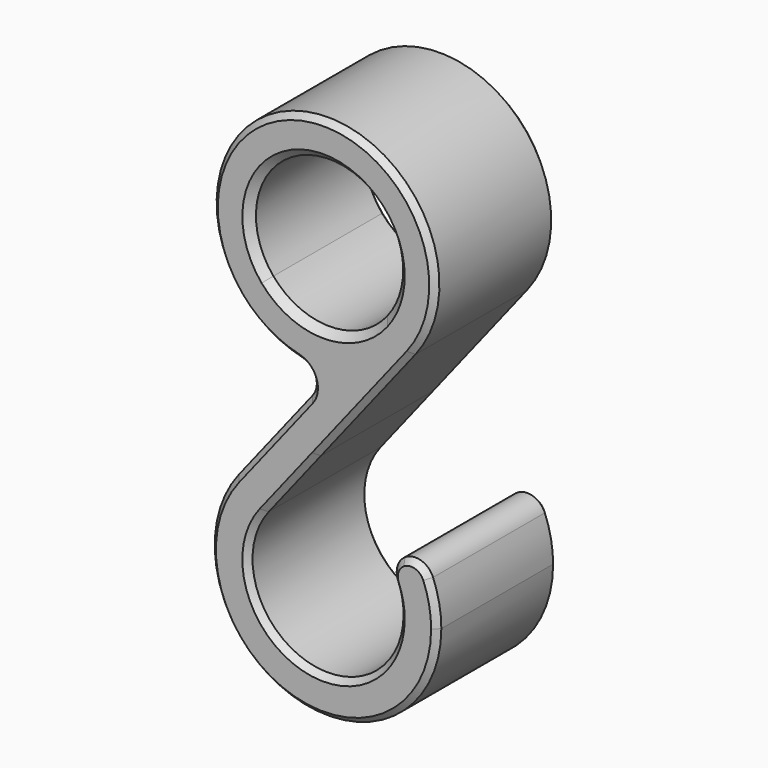
from build123d import *

# Parameters (mm, degrees)
F1_DEPTH = 16
F2_R     = 1.99999
F3_SIZE  = 0.8
F4_SIZE  = 0.6


# Not quite as in the source:
# - a fillet or chamfer is up to 0.001 mm smaller than in the source, because OpenCascade refuses the exact size


with BuildPart() as f1:
    # F0 (on Front) → F1 (new body)
    with BuildSketch(Plane.XZ):
        with BuildLine():
            ThreePointArc((7.8, 0), (7.3700465154, -2.5539017916), (6.1275860612, -4.82625))
            Line((6.1275860612, -4.82625), (0.648940015, -11.7821422864))
            ThreePointArc((0.648940015, -11.7821422864), (5.4420247731, -10.4701655368), (9.2699378875, -7.30125))
            ThreePointArc((9.2699378875, -7.30125), (11.1495575489, -3.8635950181), (11.8, 0))
            ThreePointArc((11.8, 0), (-4.0644802866, 11.0779059393), (-9, -7.6315136113))
            Line((-9, -7.6315136113), (-5.9491525424, -5.0445598448))
            ThreePointArc((-5.9491525424, -5.0445598448), (-2.6866903589, 7.322683587), (7.8, 0))
        make_face()
        with BuildLine():
            ThreePointArc((9.2699378875, -7.30125), (5.4420247731, -10.4701655368), (0.648940015, -11.7821422864))
            Line((0.648940015, -11.7821422864), (-9.4270554788, -24.575))
            ThreePointArc((-9.4270554788, -24.575), (-5.5744413376, -21.3733540676), (-0.7504354082, -20.0234877073))
            Line((-0.7504354082, -20.0234877073), (9.2699378875, -7.30125))
        make_face()
        with BuildLine():
            ThreePointArc((-0.7504354082, -20.0234877073), (-5.5744413376, -21.3733540676), (-9.4270554788, -24.575))
            ThreePointArc((-9.4270554788, -24.575), (-3.9290796794, -43.3385331006), (12, -32))
            ThreePointArc((12, -32), (11.4891252931, -28.5358983849), (10, -25.3667504193))
            Line((10, -25.3667504193), (6.6666666667, -27.5778336129))
            ThreePointArc((6.6666666667, -27.5778336129), (7.6594168621, -29.6905989232), (8, -32))
            ThreePointArc((8, -32), (-2.619386453, -39.559022067), (-6.2847036525, -27.05))
            Line((-6.2847036525, -27.05), (-0.7504354082, -20.0234877073))
        make_face()
        with BuildLine():
            Line((0.648940015, -11.7821422864), (6.1275860612, -4.82625))
            ThreePointArc((6.1275860612, -4.82625), (0.1409766904, -7.7987258942), (-5.9491525424, -5.0445598448))
            Line((-5.9491525424, -5.0445598448), (-9, -7.6315136113))
            ThreePointArc((-9, -7.6315136113), (-4.6628296471, -10.8396503487), (0.648940015, -11.7821422864))
        make_face()
    extrude(amount=F1_DEPTH)

    # F2 (radius 2 in the source; OpenCascade refuses exactly that, so slightly less here)
    f2_edges = [f1.edges().sort_by_distance(p)[0] for p in [
        (6.127586, -8, -4.82625),
        (9.269938, -8, -7.30125),
        (10, -8, -25.36675),
        (6.666667, -8, -27.577834),
        (0.64894, -8, -11.782142),
    ]]
    fillet(f2_edges, radius=F2_R)

    # F3
    f3_edges = [f1.edges().sort_by_distance(p)[0] for p in [
        (-6.127586, -16, 4.82625),
        (-6.127586, 0, 4.82625),
    ]]
    chamfer(f3_edges, length=F3_SIZE)

    # F4
    f4_edges = [f1.edges().sort_by_distance(p)[0] for p in [
        (-3.880931, -16, 11.143535),
        (1.492617, 0, -17.175625),
        (-5.523718, 0, -19.619177),
        (-1.302823, 0, -12.768079),
        (-1.69128, 0, -43.880218),
        (-3.880931, 0, 11.143535),
        (9.862297, 0, -26.340194),
        (8.164968, 0, -26.583973),
        (-1.127522, 0, -39.920145),
        (7.360063, 0, -27.658852),
        (-5.523718, -16, -19.619177),
        (-1.302823, -16, -12.768079),
        (-1.69128, -16, -43.880218),
        (9.862297, -16, -26.340194),
        (1.492617, -16, -17.175625),
        (8.164968, -16, -26.583973),
        (-1.127522, -16, -39.920145),
        (7.360063, -16, -27.658852),
    ]]
    chamfer(f4_edges, length=F4_SIZE)


solid = f1.part
